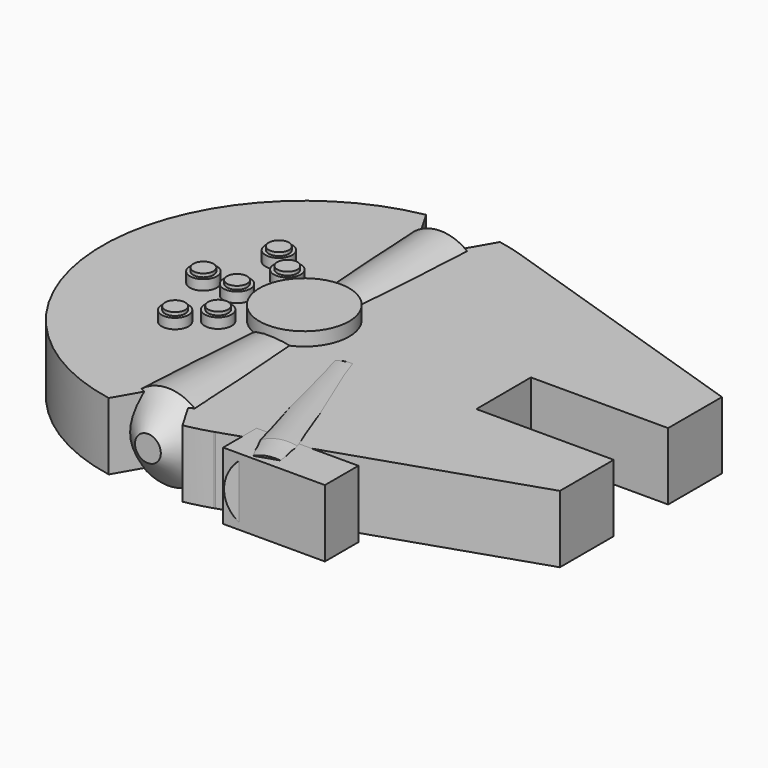
from build123d import *

# Parameters (mm, degrees)
F1_DEPTH       = 25.4
F2_R           = 16.9431619962
F3_DEPTH       = 30.48
F4_R           = 3.81
F5_DEPTH       = 30.48
F4_R_2         = 5.08
F6_DEPTH       = 29.21
F7_R           = 13.97
F8_DEPTH       = 64.2778724432
F8_TAPER       = -2
F8_DEPTH_BACK  = 64.2874
F8_TAPER_BACK  = -2
F9_R           = 16.214632767
F10_DEPTH      = 9.5203537494
F10_TAPER      = 50
F13_R          = 13.97
F14_DEPTH      = 55.0323948264
F14_TAPER      = 1
F14_DEPTH_BACK = 10.3563647717
F14_TAPER_BACK = 3
F15_W          = 38.4266898036
F15_H          = 15.8058255911
F16_DEPTH      = 25.4


with BuildPart() as f1:
    # F0 (on Top) → F1 (new body)
    with BuildSketch(Plane.XY):
        with BuildLine():
            Line((75.1342132454, -12.7), (75.0606149769, 13.1279883946))
            ThreePointArc((75.0606149769, 13.1279883946), (57.6244550994, 49.8584212997), (23.7821076654, 72.3937245553))
            ThreePointArc((23.7821076654, 72.3937245553), (18.8952117411, 73.8201258009), (13.9239792282, 74.9170394667))
            Line((13.9239792282, 74.9170394667), (0, 50.8))
            Line((0, 50.8), (-13.9239792282, 74.9170394667))
            ThreePointArc((-13.9239792282, 74.9170394667), (-76.2, 0), (-13.9239792282, -74.9170394667))
            Line((-13.9239792282, -74.9170394667), (0, -50.8))
            Line((0, -50.8), (13.9239792282, -74.9170394667))
            ThreePointArc((13.9239792282, -74.9170394667), (18.8952117411, -73.8201258009), (23.7821076654, -72.3937245553))
            Line((23.7821076654, -72.3937245553), (24.2691676459, -72.2319008595))
            ThreePointArc((24.2691676459, -72.2319008595), (57.9333223468, -49.4991935476), (75.1342132454, -12.7))
        make_face()
        with BuildLine():
            ThreePointArc((23.7821076654, 72.3937245553), (57.6244550994, 49.8584212997), (75.0606149769, 13.1279883946))
            Line((75.0606149769, 13.1279883946), (126.8708166217, 13.1279883946))
            Line((126.8708166217, 13.1279883946), (126.8708166217, 38.5279883946))
            Line((126.8708166217, 38.5279883946), (23.7821076654, 72.3937245553))
        make_face()
        with BuildLine():
            Line((127, -12.7), (75.1342132454, -12.7))
            ThreePointArc((75.1342132454, -12.7), (57.9333223468, -49.4991935476), (24.2691676459, -72.2319008595))
            Line((24.2691676459, -72.2319008595), (127, -38.1))
            Line((127, -38.1), (127, -12.7))
        make_face()
        with BuildLine():
            ThreePointArc((23.7821076654, -72.3937245553), (24.0257738998, -72.3132227778), (24.2691676459, -72.2319008595))
            Line((24.2691676459, -72.2319008595), (23.7821076654, -72.3937245553))
        make_face()
    extrude(amount=F1_DEPTH)

    # F2 (on Top) → F3 (join)
    with BuildSketch(Plane.XY):
        Circle(F2_R)
    extrude(amount=F3_DEPTH)


with BuildPart() as f5:
    # F4 (on Top) → F5 (new body)
    with BuildSketch(Plane.XY):
        with Locations((-19.4575288552, 16.326805286)):
            Circle(F4_R)
    extrude(amount=F5_DEPTH)


with BuildPart() as f5b:
    # F4 (on Top) → F5, piece 2 (new body)
    with BuildSketch(Plane.XY):
        with Locations((-29.1862932828, 24.4902079291)):
            Circle(F4_R)
    extrude(amount=F5_DEPTH)


with BuildPart() as f5c:
    # F4 (on Top) → F5, piece 3 (new body)
    with BuildSketch(Plane.XY):
        with Locations((-38.1, 0)):
            Circle(F4_R)
    extrude(amount=F5_DEPTH)


with BuildPart() as f5d:
    # F4 (on Top) → F5, piece 4 (new body)
    with BuildSketch(Plane.XY):
        with BuildLine():
            ThreePointArc((-29.21, 0), (-25.4, -3.81), (-21.59, 0))
            ThreePointArc((-21.59, 0), (-25.4, 3.81), (-29.21, 0))
        make_face()
    extrude(amount=F5_DEPTH)


with BuildPart() as f5e:
    # F4 (on Top) → F5, piece 5 (new body)
    with BuildSketch(Plane.XY):
        with Locations((-19.4575288552, -16.326805286)):
            Circle(F4_R)
    extrude(amount=F5_DEPTH)


with BuildPart() as f5f:
    # F4 (on Top) → F5, piece 6 (new body)
    with BuildSketch(Plane.XY):
        with Locations((-29.1862932828, -24.4902079291)):
            Circle(F4_R)
    extrude(amount=F5_DEPTH)


with BuildPart() as f6:
    # F4 (on Top) → F6 (new body)
    with BuildSketch(Plane.XY):
        with Locations((-29.1862932828, -24.4902079291)):
            Circle(F4_R_2)
        with Locations((-29.1862932828, -24.4902079291)):
            Circle(F4_R, mode=Mode.SUBTRACT)
    extrude(amount=F6_DEPTH)


with BuildPart() as f6b:
    # F4 (on Top) → F6, piece 2 (new body)
    with BuildSketch(Plane.XY):
        with Locations((-19.4575288552, -16.326805286)):
            Circle(F4_R_2)
        with Locations((-19.4575288552, -16.326805286)):
            Circle(F4_R, mode=Mode.SUBTRACT)
    extrude(amount=F6_DEPTH)


with BuildPart() as f6c:
    # F4 (on Top) → F6, piece 3 (new body)
    with BuildSketch(Plane.XY):
        with Locations((-25.4, 0)):
            Circle(F4_R_2)
        with BuildLine():
            ThreePointArc((-29.21, 0), (-25.4, 3.81), (-21.59, 0))
            ThreePointArc((-21.59, 0), (-25.4, -3.81), (-29.21, 0))
        make_face(mode=Mode.SUBTRACT)
    extrude(amount=F6_DEPTH)


with BuildPart() as f6d:
    # F4 (on Top) → F6, piece 4 (new body)
    with BuildSketch(Plane.XY):
        with Locations((-38.1, 0)):
            Circle(F4_R_2)
        with Locations((-38.1, 0)):
            Circle(F4_R, mode=Mode.SUBTRACT)
    extrude(amount=F6_DEPTH)


with BuildPart() as f6e:
    # F4 (on Top) → F6, piece 5 (new body)
    with BuildSketch(Plane.XY):
        with Locations((-19.4575288552, 16.326805286)):
            Circle(F4_R_2)
        with Locations((-19.4575288552, 16.326805286)):
            Circle(F4_R, mode=Mode.SUBTRACT)
    extrude(amount=F6_DEPTH)


with BuildPart() as f6f:
    # F4 (on Top) → F6, piece 6 (new body)
    with BuildSketch(Plane.XY):
        with Locations((-29.1862932828, 24.4902079291)):
            Circle(F4_R_2)
        with Locations((-29.1862932828, 24.4902079291)):
            Circle(F4_R, mode=Mode.SUBTRACT)
    extrude(amount=F6_DEPTH)


with BuildPart() as f8:
    # F7 (on Front) → F8 (new body, two sides)
    with BuildSketch(Plane.XZ) as f8_sk:
        with Locations((0, 12.7)):
            Circle(F7_R)
    extrude(amount=F8_DEPTH, taper=F8_TAPER)
    extrude(f8_sk.sketch, amount=-F8_DEPTH_BACK, taper=F8_TAPER_BACK)


with BuildPart() as f10:
    # F9 (on face) → F10 (new body)
    with BuildSketch(Plane.XZ.offset(64.2778724432)):
        with Locations((0, 12.7)):
            Circle(F9_R)
    extrude(amount=F10_DEPTH, taper=F10_TAPER)


with BuildPart() as f11_1:
    # F11: instance of F10
    add(f10.part.mirror(Plane.XZ))


with BuildPart() as f14:
    # F13 (on offset) → F14 (new body, two sides)
    with BuildSketch(Plane(origin=(24.0256376556, -72.3128127074, 0), x_dir=(0.9489924249, 0.3152988701, 0), z_dir=(0.3152988701, -0.9489924249, 0))) as f14_sk:
        with Locations((20.1903004199, 12.7)):
            Circle(F13_R)
    extrude(amount=-F14_DEPTH, taper=F14_TAPER)
    extrude(f14_sk.sketch, amount=F14_DEPTH_BACK, taper=F14_TAPER_BACK)


with BuildPart() as f16:
    # F15 (on Top) → F16 (new body)
    with BuildSketch(Plane.XY):
        with Locations((51.3752065599, -70.6009492278)):
            Rectangle(F15_W, F15_H)
    extrude(amount=F16_DEPTH)


solid = Compound([f1.part, f5.part, f5b.part, f5c.part, f5d.part, f5e.part, f5f.part, f6.part, f6b.part, f6c.part, f6d.part, f6e.part, f6f.part, f8.part, f10.part, f11_1.part, f14.part, f16.part])
